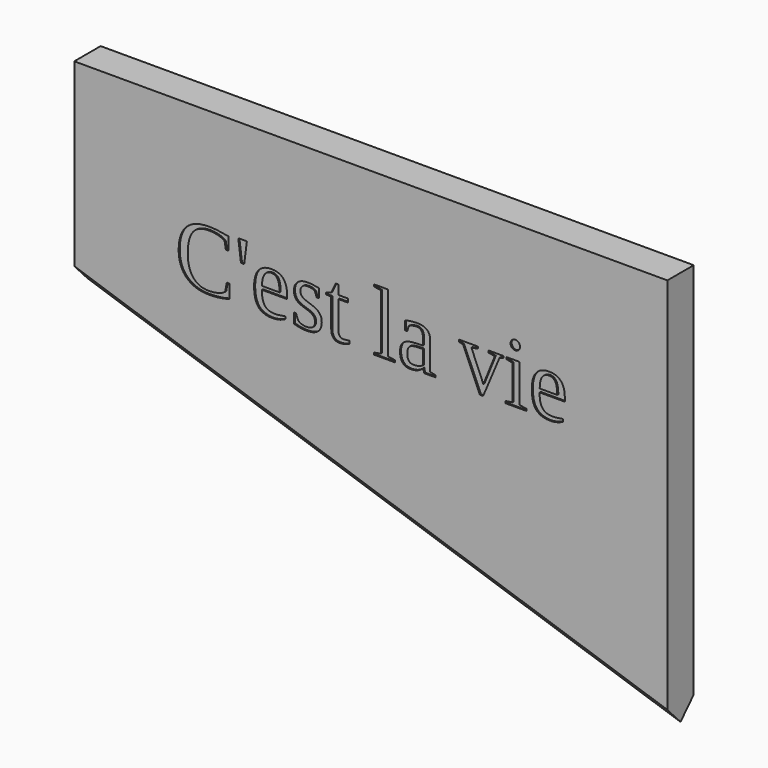
from build123d import *

# Parameters (mm, degrees)
F1_DEPTH     = 6.35
F2_SIZE      = 3.17499
F3_TEXT_SIZE = 17.2033300409
F4_DEPTH     = 0.254


# Not quite as in the source:
# - a fillet or chamfer is up to 0.001 mm smaller than in the source, because OpenCascade refuses the exact size
# - Text() gives the source's letters only with a copy of the font that has no kerning and outlines rounded to 1/6400 em; it was checked with that copy


with BuildPart() as f1:
    # F0 (on Front) → F1 (new body)
    with BuildSketch(Plane.XZ):
        Polygon((57.15, 38.1), (-57.15, 38.1), (-57.15, 0), (57.15, -38.1), align=None)
    extrude(amount=F1_DEPTH)

    # F2 (size 3.175 in the source; OpenCascade refuses exactly that, so slightly less here)
    f2_edges = [f1.edges().sort_by_distance(p)[0] for p in [
        (0, -6.35, -19.05),
        (0, 0, -19.05),
    ]]
    chamfer(f2_edges, length=F2_SIZE)

    # F3 (on face) → F4 (cut)
    with BuildSketch(Plane.XZ.offset(6.35)):
        with Locations((-37.7380049485, 7.1113246044)):
            Text("C'est la vie", F3_TEXT_SIZE, font='Tinos', text_align=(TextAlign.LEFT, TextAlign.BOTTOM))
    extrude(amount=-F4_DEPTH, mode=Mode.SUBTRACT)


solid = f1.part
